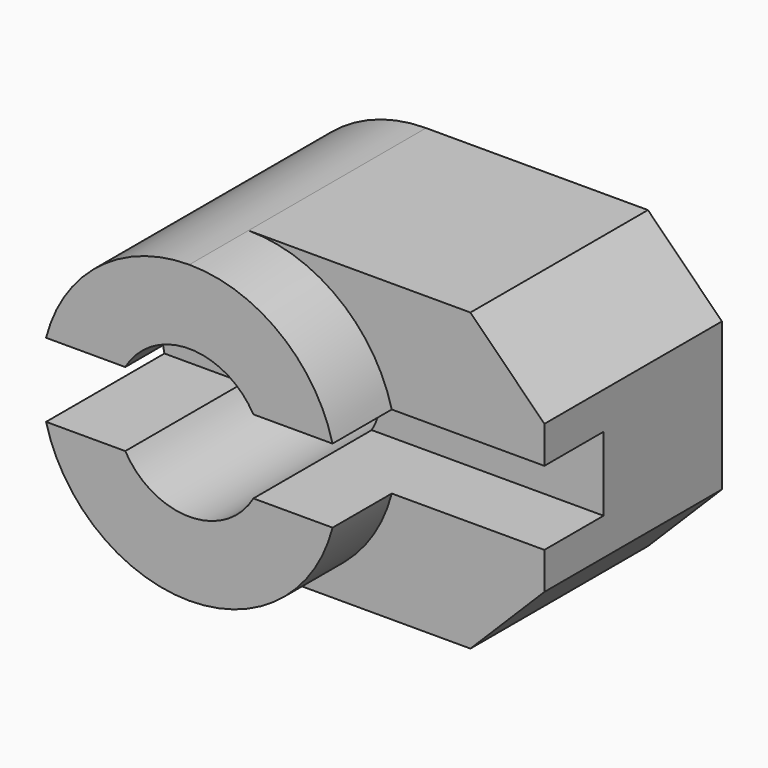
from build123d import *

# Parameters (mm, degrees)
F1_DEPTH = 15
F2_DEPTH = 10
F3_DEPTH = 15
F4_DEPTH = 10
F5_DEPTH = 20
F6_DEPTH = 10


with BuildPart() as f1:
    # F0 (on Front) → F1 (new body)
    with BuildSketch(Plane.XZ):
        with BuildLine():
            ThreePointArc((0, 10), (6.123724357, 7.9056941504), (9.6824583655, 2.5))
            Line((9.6824583655, 2.5), (20, 2.5))
            Line((20, 2.5), (20, 5))
            Line((20, 5), (15, 10))
            Line((15, 10), (0, 10))
        make_face()
    extrude(amount=F1_DEPTH)

    # F0 (on Front) → F2 (join)
    with BuildSketch(Plane.XZ):
        with BuildLine():
            Line((20, 2.5), (9.6824583655, 2.5))
            ThreePointArc((9.6824583655, 2.5), (9.9202969627, 1.2600429248), (10, 0))
            ThreePointArc((10, 0), (9.9202969627, -1.2600429248), (9.6824583655, -2.5))
            Line((9.6824583655, -2.5), (20, -2.5))
            Line((20, -2.5), (20, 2.5))
        make_face()
    extrude(amount=F2_DEPTH)

    # F0 (on Front) → F3 (join)
    with BuildSketch(Plane.XZ):
        with BuildLine():
            Line((20, -2.5), (9.6824583655, -2.5))
            ThreePointArc((9.6824583655, -2.5), (6.123724357, -7.9056941504), (0, -10))
            Line((0, -10), (15, -10))
            Line((15, -10), (20, -5))
            Line((20, -5), (20, -2.5))
        make_face()
    extrude(amount=F3_DEPTH)

    # F0 (on Front) → F4 (join)
    with BuildSketch(Plane.XZ):
        with BuildLine():
            ThreePointArc((4.3301270189, 2.5), (4.8296291314, 1.2940952255), (5, 0))
            ThreePointArc((5, 0), (4.8296291314, -1.2940952255), (4.3301270189, -2.5))
            Line((4.3301270189, -2.5), (9.6824583655, -2.5))
            ThreePointArc((9.6824583655, -2.5), (9.9202969627, -1.2600429248), (10, 0))
            ThreePointArc((10, 0), (9.9202969627, 1.2600429248), (9.6824583655, 2.5))
            Line((9.6824583655, 2.5), (4.3301270189, 2.5))
        make_face()
    extrude(amount=F4_DEPTH)

    # F0 (on Front) → F5 (join)
    with BuildSketch(Plane.XZ):
        with BuildLine():
            ThreePointArc((-4.3301270189, 2.5), (0, 5), (4.3301270189, 2.5))
            Line((4.3301270189, 2.5), (9.6824583655, 2.5))
            ThreePointArc((9.6824583655, 2.5), (6.123724357, 7.9056941504), (0, 10))
            ThreePointArc((0, 10), (-6.123724357, 7.9056941504), (-9.6824583655, 2.5))
            Line((-9.6824583655, 2.5), (-4.3301270189, 2.5))
        make_face()
        with BuildLine():
            Line((9.6824583655, -2.5), (4.3301270189, -2.5))
            ThreePointArc((4.3301270189, -2.5), (0, -5), (-4.3301270189, -2.5))
            Line((-4.3301270189, -2.5), (-9.6824583655, -2.5))
            ThreePointArc((-9.6824583655, -2.5), (-6.123724357, -7.9056941504), (0, -10))
            ThreePointArc((0, -10), (6.123724357, -7.9056941504), (9.6824583655, -2.5))
        make_face()
    extrude(amount=F5_DEPTH)

    # F0 (on Front) → F6 (join)
    with BuildSketch(Plane.XZ):
        with BuildLine():
            ThreePointArc((-4.3301270189, -2.5), (-5, 0), (-4.3301270189, 2.5))
            Line((-4.3301270189, 2.5), (-9.6824583655, 2.5))
            ThreePointArc((-9.6824583655, 2.5), (-10, 0), (-9.6824583655, -2.5))
            Line((-9.6824583655, -2.5), (-4.3301270189, -2.5))
        make_face()
    extrude(amount=F6_DEPTH)


solid = f1.part
